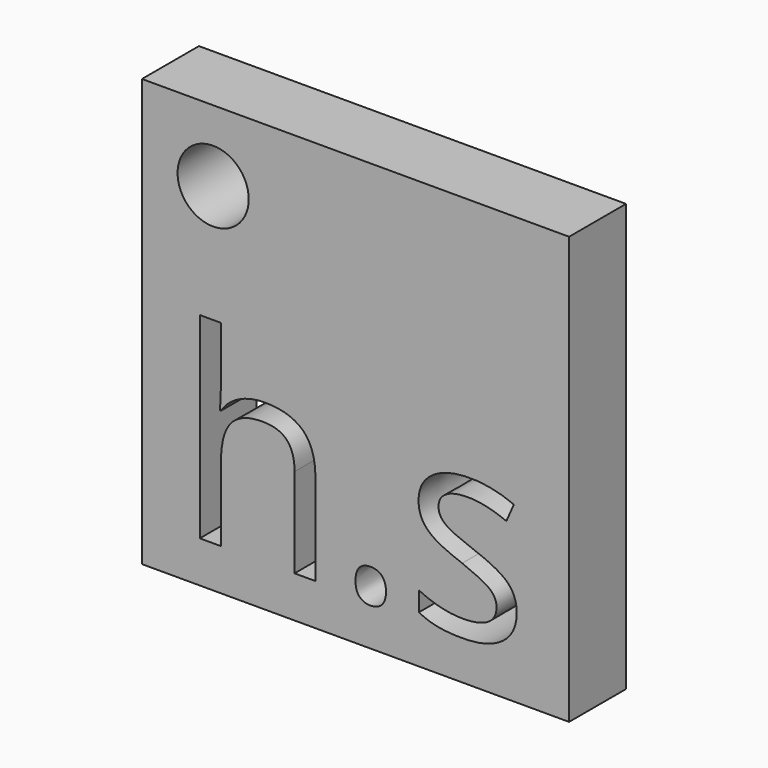
from build123d import *

# Parameters (mm, degrees)
F0_W         = 30
F0_H         = 30
F0_R         = 2.5
F1_DEPTH     = 5
F2_TEXT_SIZE = 18.1714934696
F3_DEPTH     = 5.001


# Not quite as in the source:
# - a feature names something its author has since deleted; it is built from what else it names
# - Text() gives the source's letters only with a copy of the font that has no kerning and outlines rounded to 1/6400 em; it was checked with that copy


with BuildPart() as f1:
    # F0 (on Front) → F1 (new body)
    with BuildSketch(Plane.XZ):
        with Locations((15, 15)):
            Rectangle(F0_W, F0_H)
        with Locations((5, 25)):
            Circle(F0_R, mode=Mode.SUBTRACT)
    extrude(amount=F1_DEPTH)

    # F2 (on face) → F3 (cut, through all)
    with BuildSketch(Plane.XZ.offset(5)):
        with Locations((2.5, 2.9165247019)):
            Text('h.s', F2_TEXT_SIZE, font='Open Sans', text_align=(TextAlign.LEFT, TextAlign.BOTTOM))
    extrude(amount=-F3_DEPTH, mode=Mode.SUBTRACT)


solid = f1.part
